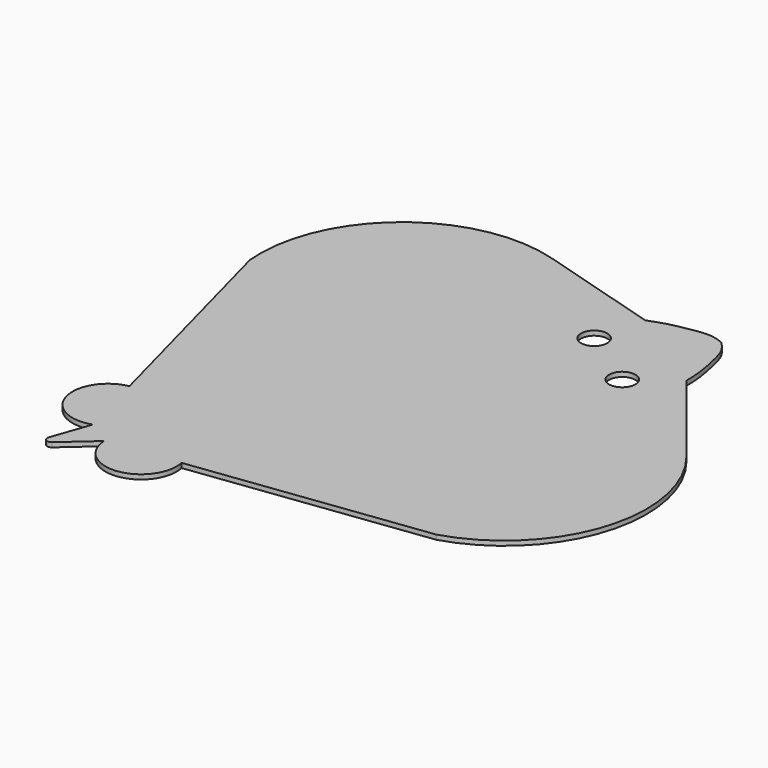
from build123d import *

# Parameters (mm, degrees)
F0_R     = 9.082794509
F1_DEPTH = 3.175
F2_SCALE = 0.8


# Not quite as in the source:
# - a feature names something its author has since deleted; it is built from what else it names


with BuildPart() as f1:
    # F0 (on Top) → F1 (new body)
    with BuildSketch(Plane.XY):
        with BuildLine():
            Line((190.1853488741, -177.0173265019), (349.6757983606, -156.6053567409))
            ThreePointArc((349.6757983606, -156.6053567409), (414.8838780797, -91.7557523294), (397.7330321915, -1.4041428346))
            Line((397.7330321915, -1.4041428346), (342.5045750448, 67.5291355358))
            add(Edge.make_bspline(
                [(329.4549969886, 114.1704269865), (331.5452640948, 111.8836468118), (336.0081220097, 107.0012205554), (339.0892090613, 95.2737066428), (342.2686372384, 79.5699362539), (342.4299296899, 71.3385709799), (342.5045750448, 67.5291355358)],
                knots=[0, 0, 0, 0, 0.2181778066, 0.4658239841, 0.7527859619, 1, 1, 1, 1], degree=3))
            add(Edge.make_bspline(
                [(329.4549969886, 114.1704269865), (326.548311382, 115.2426951096), (320.3423462083, 117.5320581607), (308.3194887471, 115.9577079905), (292.5774945842, 112.9732838027), (284.8943646943, 110.0150910055), (281.3386498949, 108.6460538997)],
                knots=[0, 0, 0, 0, 0.2181778066, 0.4658239841, 0.7527859619, 1, 1, 1, 1], degree=3))
            Line((281.3386498949, 108.6460538997), (196.6563418366, 133.7634989848))
            ThreePointArc((196.6563418366, 133.7634989848), (106.5159411756, 115.5351413614), (71.0829640293, 30.6701368923))
            Line((71.0829640293, 30.6701368923), (112.3931918139, -124.7239333526))
            Line((112.3931918139, -124.7239333526), (124.9610056376, -171.9994834736))
            Line((124.9610056376, -171.9994834736), (128.3971803048, -184.9251243198))
            Line((128.3971803048, -184.9251243198), (141.6635569768, -183.2272616556))
            Line((141.6635569768, -183.2272616556), (190.1853488741, -177.0173265019))
        make_face()
        with Locations((314.69919144, 47.0405749589)):
            Circle(F0_R, mode=Mode.SUBTRACT)
        with Locations((272.863497229, 75.1633380718)):
            Circle(F0_R, mode=Mode.SUBTRACT)
        with BuildLine():
            ThreePointArc((112.3931918139, -124.7239333526), (93.1968044826, -155.1354338039), (124.9610056376, -171.9994834736))
            Line((124.9610056376, -171.9994834736), (112.3931918139, -124.7239333526))
        make_face()
        with BuildLine():
            ThreePointArc((141.6635569768, -183.2272616556), (169.2714467636, -206.2742802869), (190.1853488741, -177.0173265019))
            Line((190.1853488741, -177.0173265019), (141.6635569768, -183.2272616556))
        make_face()
        with BuildLine():
            Line((120.3224166543, -196.9372207683), (128.3971803048, -184.9251243198))
            Line((128.3971803048, -184.9251243198), (124.9610056376, -171.9994834736))
            Line((124.9610056376, -171.9994834736), (115.7260780635, -198.4687475134))
            ThreePointArc((115.7260780635, -198.4687475134), (117.6479584787, -196.5736854806), (120.3224166543, -196.9372207683))
        make_face()
        with BuildLine():
            Line((120.6394586436, -201.7716170066), (141.6635569768, -183.2272616556))
            Line((141.6635569768, -183.2272616556), (128.3971803048, -184.9251243198))
            Line((128.3971803048, -184.9251243198), (120.3224166543, -196.9372207683))
            ThreePointArc((120.3224166543, -196.9372207683), (121.6687259476, -199.2765231696), (120.6394586436, -201.7716170066))
        make_face()
        with BuildLine():
            ThreePointArc((116.9081491924, -202.0163180432), (118.8155291594, -202.53021243), (120.6394586436, -201.7716170066))
            ThreePointArc((120.6394586436, -201.7716170066), (121.6687259476, -199.2765231696), (120.3224166543, -196.9372207683))
            Line((120.3224166543, -196.9372207683), (116.9081491924, -202.0163180432))
        make_face()
        with BuildLine():
            Line((116.9081491924, -202.0163180432), (120.3224166543, -196.9372207683))
            ThreePointArc((120.3224166543, -196.9372207683), (117.6479584787, -196.5736854806), (115.7260780635, -198.4687475134))
            ThreePointArc((115.7260780635, -198.4687475134), (115.7121989982, -200.4440938504), (116.9081491924, -202.0163180432))
        make_face()
    extrude(amount=F1_DEPTH)


with BuildPart() as f1_1:
    # F2: moved
    add(f1.part.scale(F2_SCALE).moved(Location((51.3425254966, 2.2402065434, 0))))


solid = f1_1.part
